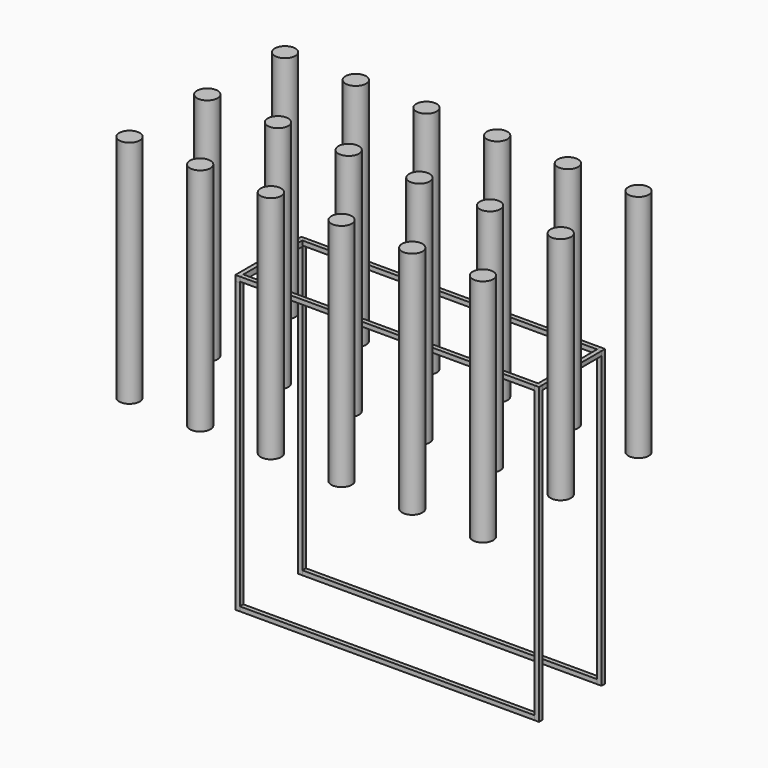
from build123d import *

# Parameters (mm, degrees)
F0_W      = 30
F0_H      = 30
F1_DEPTH  = 2000
F2_W      = 30
F2_H      = 30
F3_DEPTH  = 2000
F4_W      = 30
F4_H      = 30
F5_DEPTH  = 2000
F6_W      = 30
F6_H      = 37.5192165375
F7_DEPTH  = 530
F8_W      = 30
F8_H      = 30
F9_DEPTH  = 500
F12_R     = 69.6234629817
F13_DEPTH = 1559.8455667496


with BuildPart() as f1:
    # F0 (on Top) → F1 (new body)
    with BuildSketch(Plane.XY):
        with Locations((-1015, 265)):
            Rectangle(F0_W, F0_H)
    extrude(amount=F1_DEPTH)


with BuildPart() as f1b:
    # F0 (on Top) → F1, piece 2 (new body)
    with BuildSketch(Plane.XY):
        with Locations((1015, 265)):
            Rectangle(F0_W, F0_H)
    extrude(amount=F1_DEPTH)


with BuildPart() as f1c:
    # F0 (on Top) → F1, piece 3 (new body)
    with BuildSketch(Plane.XY):
        with Locations((-1015, -265)):
            Rectangle(F0_W, F0_H)
    extrude(amount=F1_DEPTH)


with BuildPart() as f1d:
    # F0 (on Top) → F1, piece 4 (new body)
    with BuildSketch(Plane.XY):
        with Locations((1015, -265)):
            Rectangle(F0_W, F0_H)
    extrude(amount=F1_DEPTH)


with BuildPart() as f3:
    # F2 (on face) → F3 (new body, through all)
    with BuildSketch(Plane.YZ.offset(-1000)):
        with Locations((265, 15)):
            Rectangle(F2_W, F2_H)
    extrude(amount=F3_DEPTH)


with BuildPart() as f3b:
    # F2 (on face) → F3, piece 2 (new body, through all)
    with BuildSketch(Plane.YZ.offset(-1000)):
        with Locations((-265, 15)):
            Rectangle(F2_W, F2_H)
    extrude(amount=F3_DEPTH)


with BuildPart() as f5:
    # F4 (on face) → F5 (new body, through all)
    with BuildSketch(Plane.YZ.offset(-1000)):
        with Locations((-265, 1985)):
            Rectangle(F4_W, F4_H)
    extrude(amount=F5_DEPTH)


with BuildPart() as f5b:
    # F4 (on face) → F5, piece 2 (new body, through all)
    with BuildSketch(Plane.YZ.offset(-1000)):
        with Locations((265, 1985)):
            Rectangle(F4_W, F4_H)
    extrude(amount=F5_DEPTH)


with BuildPart() as f7:
    # F6 (on face) → F7 (new body, through all)
    with BuildSketch(Plane.XZ.offset(280)):
        with Locations((-1015, 1981.2403917313)):
            Rectangle(F6_W, F6_H)
    extrude(amount=-F7_DEPTH)


with BuildPart() as f9:
    # F8 (on face) → F9 (new body)
    with BuildSketch(Plane.XZ.offset(-250)):
        with Locations((1015, 1985)):
            Rectangle(F8_W, F8_H)
    extrude(amount=F9_DEPTH)


with BuildPart() as f13:
    # F12 (on face) → F13 (new body)
    with BuildSketch(Plane(origin=(0, 0, 1760.2030038834), x_dir=(1, 0, 0), z_dir=(0, 0, -1))):
        with Locations((-836.7166519165, 100.225508213)):
            Circle(F12_R)
    extrude(amount=-F13_DEPTH)


with BuildPart() as f13b:
    # F12 (on face) → F13, piece 2 (new body)
    with BuildSketch(Plane(origin=(0, 0, 1760.2030038834), x_dir=(1, 0, 0), z_dir=(0, 0, -1))):
        with Locations((-855.7178974152, 736.188262701)):
            Circle(F12_R)
    extrude(amount=-F13_DEPTH)


with BuildPart() as f13c:
    # F12 (on face) → F13, piece 3 (new body)
    with BuildSketch(Plane(origin=(0, 0, 1760.2030038834), x_dir=(1, 0, 0), z_dir=(0, 0, -1))):
        with Locations((-345.4257249832, 114.8418784142)):
            Circle(F12_R)
    extrude(amount=-F13_DEPTH)


with BuildPart() as f13d:
    # F12 (on face) → F13, piece 4 (new body)
    with BuildSketch(Plane(origin=(0, 0, 1760.2030038834), x_dir=(1, 0, 0), z_dir=(0, 0, -1))):
        with Locations((-364.4269704819, 750.8046329021)):
            Circle(F12_R)
    extrude(amount=-F13_DEPTH)


with BuildPart() as f13e:
    # F12 (on face) → F13, piece 5 (new body)
    with BuildSketch(Plane(origin=(0, 0, 1760.2030038834), x_dir=(1, 0, 0), z_dir=(0, 0, -1))):
        with Locations((145.8652019501, 129.4582486153)):
            Circle(F12_R)
    extrude(amount=-F13_DEPTH)


with BuildPart() as f13f:
    # F12 (on face) → F13, piece 6 (new body)
    with BuildSketch(Plane(origin=(0, 0, 1760.2030038834), x_dir=(1, 0, 0), z_dir=(0, 0, -1))):
        with Locations((126.8639564514, 765.4210031033)):
            Circle(F12_R)
    extrude(amount=-F13_DEPTH)


with BuildPart() as f13g:
    # F12 (on face) → F13, piece 7 (new body)
    with BuildSketch(Plane(origin=(0, 0, 1760.2030038834), x_dir=(1, 0, 0), z_dir=(0, 0, -1))):
        with Locations((-874.7191429138, 1372.151017189)):
            Circle(F12_R)
    extrude(amount=-F13_DEPTH)


with BuildPart() as f13h:
    # F12 (on face) → F13, piece 8 (new body)
    with BuildSketch(Plane(origin=(0, 0, 1760.2030038834), x_dir=(1, 0, 0), z_dir=(0, 0, -1))):
        with Locations((-383.4282159805, 1386.7673873901)):
            Circle(F12_R)
    extrude(amount=-F13_DEPTH)


with BuildPart() as f13i:
    # F12 (on face) → F13, piece 9 (new body)
    with BuildSketch(Plane(origin=(0, 0, 1760.2030038834), x_dir=(1, 0, 0), z_dir=(0, 0, -1))):
        with Locations((107.8627109528, 1401.3837575912)):
            Circle(F12_R)
    extrude(amount=-F13_DEPTH)


with BuildPart() as f13j:
    # F12 (on face) → F13, piece 10 (new body)
    with BuildSketch(Plane(origin=(0, 0, 1760.2030038834), x_dir=(1, 0, 0), z_dir=(0, 0, -1))):
        with Locations((637.1561288834, 144.0746188164)):
            Circle(F12_R)
    extrude(amount=-F13_DEPTH)


with BuildPart() as f13k:
    # F12 (on face) → F13, piece 11 (new body)
    with BuildSketch(Plane(origin=(0, 0, 1760.2030038834), x_dir=(1, 0, 0), z_dir=(0, 0, -1))):
        with Locations((618.1548833847, 780.0373733044)):
            Circle(F12_R)
    extrude(amount=-F13_DEPTH)


with BuildPart() as f13l:
    # F12 (on face) → F13, piece 12 (new body)
    with BuildSketch(Plane(origin=(0, 0, 1760.2030038834), x_dir=(1, 0, 0), z_dir=(0, 0, -1))):
        with Locations((599.153637886, 1416.0001277924)):
            Circle(F12_R)
    extrude(amount=-F13_DEPTH)


with BuildPart() as f13m:
    # F12 (on face) → F13, piece 13 (new body)
    with BuildSketch(Plane(origin=(0, 0, 1760.2030038834), x_dir=(1, 0, 0), z_dir=(0, 0, -1))):
        with Locations((1128.4470558167, 158.6909890175)):
            Circle(F12_R)
    extrude(amount=-F13_DEPTH)


with BuildPart() as f13n:
    # F12 (on face) → F13, piece 14 (new body)
    with BuildSketch(Plane(origin=(0, 0, 1760.2030038834), x_dir=(1, 0, 0), z_dir=(0, 0, -1))):
        with Locations((1109.445810318, 794.6537435055)):
            Circle(F12_R)
    extrude(amount=-F13_DEPTH)


with BuildPart() as f13o:
    # F12 (on face) → F13, piece 15 (new body)
    with BuildSketch(Plane(origin=(0, 0, 1760.2030038834), x_dir=(1, 0, 0), z_dir=(0, 0, -1))):
        with Locations((1090.4445648193, 1430.6164979935)):
            Circle(F12_R)
    extrude(amount=-F13_DEPTH)


with BuildPart() as f13p:
    # F12 (on face) → F13, piece 16 (new body)
    with BuildSketch(Plane(origin=(0, 0, 1760.2030038834), x_dir=(1, 0, 0), z_dir=(0, 0, -1))):
        with Locations((1619.7379827499, 173.3073592186)):
            Circle(F12_R)
    extrude(amount=-F13_DEPTH)


with BuildPart() as f13q:
    # F12 (on face) → F13, piece 17 (new body)
    with BuildSketch(Plane(origin=(0, 0, 1760.2030038834), x_dir=(1, 0, 0), z_dir=(0, 0, -1))):
        with Locations((1600.7367372513, 809.2701137066)):
            Circle(F12_R)
    extrude(amount=-F13_DEPTH)


with BuildPart() as f13r:
    # F12 (on face) → F13, piece 18 (new body)
    with BuildSketch(Plane(origin=(0, 0, 1760.2030038834), x_dir=(1, 0, 0), z_dir=(0, 0, -1))):
        with Locations((1581.7354917526, 1445.2328681946)):
            Circle(F12_R)
    extrude(amount=-F13_DEPTH)


solid = Compound([f1.part, f1b.part, f1c.part, f1d.part, f3.part, f3b.part, f5.part, f5b.part, f7.part, f9.part, f13.part, f13b.part, f13c.part, f13d.part, f13e.part, f13f.part, f13g.part, f13h.part, f13i.part, f13j.part, f13k.part, f13l.part, f13m.part, f13n.part, f13o.part, f13p.part, f13q.part, f13r.part])
